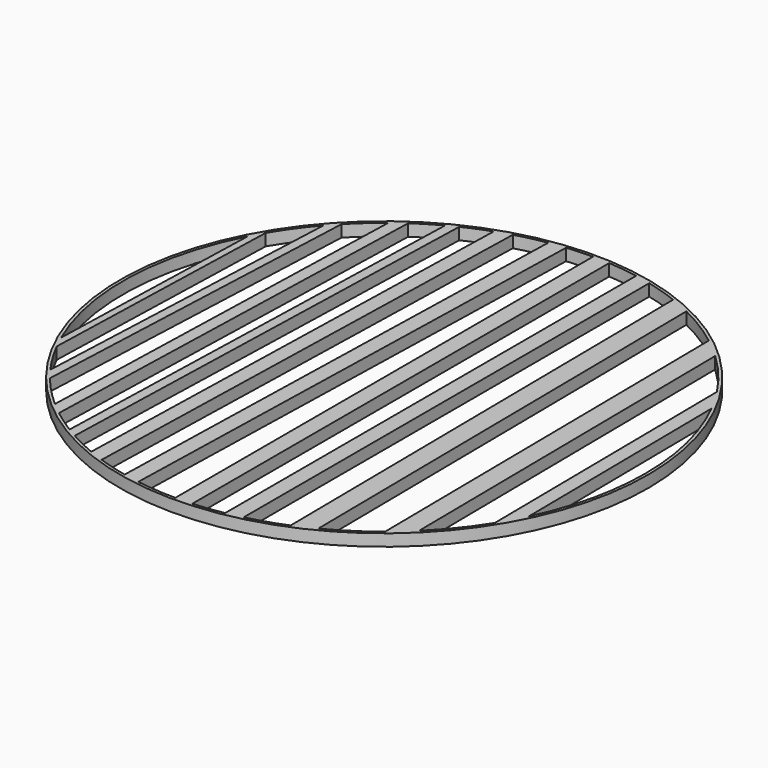
from build123d import *

# Parameters (mm, degrees)
F1_DEPTH = 20


with BuildPart() as f1:
    # F0 (on Top) → F1 (new body)
    with BuildSketch(Plane.XY):
        with BuildLine():
            Line((-270.5386970375, -346.9997311313), (-270.7217620056, -353.178039488))
            ThreePointArc((-270.7217620056, -353.178039488), (-250.9562000988, -367.4860346081), (-230.4360952891, -380.6891198707))
            Line((-230.4360952891, -380.6891198707), (-230.265657339, -374.9369641023))
            ThreePointArc((-230.2656573389, -374.9369641023), (-250.7914922543, -361.5295664436), (-270.5386970375, -346.9997311313))
        make_face()
        with BuildLine():
            ThreePointArc((-402.562994487, -177.6035908131), (-397.2206510106, -189.250507029), (-391.5414264828, -200.7369207392))
            Line((-391.5414264828, -200.7369207392), (-378.8101580312, 223.8366908537))
            ThreePointArc((-378.8101580312, 223.8366908537), (-385.1674232463, 212.7112034422), (-391.1980296982, 201.4053166136))
            Line((-391.1980296982, 201.4053166136), (-402.562994487, -177.6035908131))
        make_face()
        with BuildLine():
            ThreePointArc((-356.5130720875, -257.8728939433), (-349.3185745571, -267.5379103406), (-341.8621362052, -277.0023101514))
            Line((-341.8621362052, -277.0023101514), (-316.4372711676, 305.7244730407))
            ThreePointArc((-316.4372711676, 305.7244730407), (-324.6896849683, 296.9454638064), (-332.6986262228, 287.9437863707))
            Line((-332.6986262228, 287.9437863707), (-356.5130720875, -257.8728939433))
        make_face()
        with BuildLine():
            ThreePointArc((-290.771309932, -330.2302913429), (-280.7802245685, -338.7660925938), (-270.5386970375, -346.9997311313))
            Line((-270.5386970375, -346.9997311313), (-249.5187169425, 362.4091746843))
            ThreePointArc((-249.5187169425, 362.4091746843), (-260.22977901, 354.7963671127), (-270.708728898, 346.8670986105))
            Line((-270.708728898, 346.8670986105), (-290.771309932, -330.2302913429))
        make_face()
        with BuildLine():
            Line((-207.6622074156, 387.912886627), (-230.265657339, -374.9369641023))
            ThreePointArc((-230.2656573389, -374.9369641023), (-222.1173118779, -379.8208785258), (-213.8654246951, -384.5277364768))
            Line((-213.8654246951, -384.5277364768), (-190.7228909108, 396.5157990328))
            ThreePointArc((-190.7228909108, 396.5157990328), (-199.2389875692, 392.3057810336), (-207.6622074156, 387.912886627))
        make_face()
        with BuildLine():
            Line((-70.8738586956, 434.2544140865), (-70.7405367429, 439.341298379))
            ThreePointArc((-70.7405367429, 439.341298379), (-431.4752027521, 108.8767624889), (-270.7217620056, -353.178039488))
            Line((-270.7217620056, -353.178039488), (-270.5386970375, -346.9997311313))
            ThreePointArc((-270.5386970375, -346.9997311313), (-280.7802245685, -338.7660925938), (-290.771309932, -330.2302913429))
            ThreePointArc((-290.771309932, -330.2302913429), (-317.4343613856, -304.6890648049), (-341.8621362052, -277.0023101514))
            ThreePointArc((-341.8621362052, -277.0023101514), (-349.3185745571, -267.5379103406), (-356.5130720875, -257.8728939433))
            ThreePointArc((-356.5130720875, -257.8728939433), (-375.1166659405, -229.9727960731), (-391.5414264828, -200.7369207392))
            ThreePointArc((-391.5414264828, -200.7369207392), (-397.2206510106, -189.250507029), (-402.562994487, -177.6035908131))
            ThreePointArc((-402.562994487, -177.6035908131), (-439.8023179294, 13.187916588), (-391.1980296982, 201.4053166136))
            ThreePointArc((-391.1980296982, 201.4053166136), (-385.1674232463, 212.7112034422), (-378.8101580312, 223.8366908537))
            ThreePointArc((-378.8101580312, 223.8366908537), (-357.1954891114, 256.9268038926), (-332.6986262228, 287.9437863707))
            ThreePointArc((-332.6986262228, 287.9437863707), (-324.6896849683, 296.9454638064), (-316.4372711676, 305.7244730407))
            ThreePointArc((-316.4372711676, 305.7244730407), (-294.2928562808, 327.0958800445), (-270.708728898, 346.8670986105))
            ThreePointArc((-270.708728898, 346.8670986105), (-260.22977901, 354.7963671127), (-249.5187169425, 362.4091746843))
            ThreePointArc((-249.5187169425, 362.4091746843), (-228.9458652825, 375.7443156856), (-207.6622074156, 387.912886627))
            ThreePointArc((-207.6622074156, 387.912886627), (-199.2389875692, 392.3057810336), (-190.7228909108, 396.5157990328))
            ThreePointArc((-190.7228909108, 396.5157990328), (-169.0852127848, 406.2144640673), (-146.9564772982, 414.7334008494))
            ThreePointArc((-146.9564772982, 414.7334008494), (-134.2564645291, 419.0169468317), (-121.4318768159, 422.9116920741))
            ThreePointArc((-121.4318768159, 422.9116920741), (-96.3199787859, 429.3279185968), (-70.8738586956, 434.2544140865))
        make_face()
        with BuildLine():
            Line((-143.4181009985, -415.9702493039), (-121.4318768159, 422.9116920741))
            ThreePointArc((-121.4318768159, 422.9116920741), (-134.2564645291, 419.0169468317), (-146.9564772982, 414.7334008494))
            Line((-146.9564772982, 414.7334008494), (-168.4792645982, -406.4661577554))
            ThreePointArc((-168.4792645982, -406.4661577554), (-156.0210678261, -411.4090742733), (-143.4181009985, -415.9702493039))
        make_face()
        with BuildLine():
            ThreePointArc((-43.616286433, 437.8328671511), (-57.2730273731, 436.2565762662), (-70.8738586956, 434.2544140865))
            Line((-70.8738586956, 434.2544140865), (-93.5236465706, -429.9457262634))
            ThreePointArc((-93.5236465706, -429.9457262634), (-80.0463646466, -432.6575776603), (-66.4909418972, -434.9470710852))
            Line((-66.4909418972, -434.9470710852), (-43.616286433, 437.8328671511))
        make_face()
        with BuildLine():
            Line((0, 440), (0, -440))
            ThreePointArc((0, -440), (14.0186355194, -439.7766226827), (28.0230371971, -439.1067175372))
            Line((28.0230371971, -439.1067175372), (28.0230371971, 439.1067175372))
            ThreePointArc((28.0230371971, 439.1067175372), (14.0186355194, 439.7766226827), (0, 440))
        make_face()
        with BuildLine():
            Line((78.35839003, 432.9664683459), (78.35839003, -432.9664683459))
            ThreePointArc((78.35839003, -432.9664683459), (91.7286409393, -430.3322628289), (105.0109050122, -427.2852792088))
            Line((105.0109050122, -427.2852792088), (105.0109050122, 427.2852792088))
            ThreePointArc((105.0109050122, 427.2852792088), (91.7286409393, 430.3322628289), (78.35839003, 432.9664683459))
        make_face()
        with BuildLine():
            Line((158.8886932936, 410.3101060704), (167.7992454591, -406.7473579796))
            ThreePointArc((167.7992454591, -406.7473579796), (184.9665523772, -399.233483693), (201.798344937, -390.9954321737))
            Line((201.798344937, -390.9954321737), (193.2232359584, 395.3034038378))
            ThreePointArc((193.2232359584, 395.3034038378), (176.2157852134, 403.1724160228), (158.8886932936, 410.3101060704))
        make_face()
        with BuildLine():
            Line((268.376457209, 348.6747441613), (275.9167800325, -342.7388663348))
            ThreePointArc((275.9167800325, -342.7388663348), (292.9545944223, -328.2949978402), (309.2374568684, -313.0051042228))
            Line((309.2374568684, -313.0051042228), (302.3376646701, 319.6747355075))
            ThreePointArc((302.3376646701, 319.6747355075), (285.7252217666, 334.6058840583), (268.376457209, 348.6747441613))
        make_face()
        with BuildLine():
            Line((367.9772639554, 241.2317002633), (373.1507016006, -233.1492095096))
            ThreePointArc((373.1507016006, -233.1492095096), (385.3711791661, -212.3418335329), (396.4325833067, -190.8958011398))
            Line((396.4325833067, -190.8958011398), (392.175101476, 199.4960896417))
            ThreePointArc((392.175101476, 199.4960896417), (380.6486174495, 220.6957861714), (367.9772639554, 241.2317002633))
        make_face()
        with BuildLine():
            ThreePointArc((0, -445), (314.662517628, -314.662517628), (445, 0))
            ThreePointArc((445, 0), (288.570148447, 338.7510434306), (-70.7405367429, 439.341298379))
            Line((-70.7405367429, 439.341298379), (-70.8738586956, 434.2544140865))
            ThreePointArc((-70.8738586956, 434.2544140865), (-57.2730273731, 436.2565762662), (-43.616286433, 437.8328671511))
            ThreePointArc((-43.616286433, 437.8328671511), (-21.835045838, 439.4578828207), (0, 440))
            ThreePointArc((0, 440), (14.0186355194, 439.7766226827), (28.0230371971, 439.1067175372))
            ThreePointArc((28.0230371971, 439.1067175372), (53.2792424848, 436.7623178804), (78.35839003, 432.9664683459))
            ThreePointArc((78.35839003, 432.9664683459), (91.7286409393, 430.3322628289), (105.0109050122, 427.2852792088))
            ThreePointArc((105.0109050122, 427.2852792088), (132.2224966571, 419.663211847), (158.8886932936, 410.3101060704))
            ThreePointArc((158.8886932936, 410.3101060704), (176.2157852134, 403.1724160228), (193.2232359584, 395.3034038378))
            ThreePointArc((193.2232359584, 395.3034038378), (231.9744105691, 373.8821643795), (268.376457209, 348.6747441613))
            ThreePointArc((268.376457209, 348.6747441613), (285.7252217666, 334.6058840583), (302.3376646701, 319.6747355075))
            ThreePointArc((302.3376646701, 319.6747355075), (337.4445929766, 282.3670424658), (367.9772639554, 241.2317002633))
            ThreePointArc((367.9772639554, 241.2317002633), (380.6486174495, 220.6957861714), (392.175101476, 199.4960896417))
            ThreePointArc((392.175101476, 199.4960896417), (427.8767606738, 102.5742544467), (440, 0))
            ThreePointArc((440, 0), (428.969892099, -97.9021535643), (396.4325833067, -190.8958011398))
            ThreePointArc((396.4325833067, -190.8958011398), (385.3711791661, -212.3418335329), (373.1507016006, -233.1492095096))
            ThreePointArc((373.1507016006, -233.1492095096), (343.5224020131, -274.9406468952), (309.2374568684, -313.0051042228))
            ThreePointArc((309.2374568684, -313.0051042228), (292.9545944223, -328.2949978402), (275.9167800325, -342.7388663348))
            ThreePointArc((275.9167800325, -342.7388663348), (240.0731330091, -368.7341736362), (201.798344937, -390.9954321737))
            ThreePointArc((201.798344937, -390.9954321737), (184.9665523772, -399.233483693), (167.7992454591, -406.7473579796))
            ThreePointArc((167.7992454591, -406.7473579796), (136.7910673332, -418.1963700199), (105.0109050122, -427.2852792088))
            ThreePointArc((105.0109050122, -427.2852792088), (91.7286409393, -430.3322628289), (78.35839003, -432.9664683459))
            ThreePointArc((78.35839003, -432.9664683459), (53.2792424848, -436.7623178804), (28.0230371971, -439.1067175372))
            ThreePointArc((28.0230371971, -439.1067175372), (14.0186355194, -439.7766226827), (0, -440))
            Line((0, -440), (0, -445))
        make_face()
        with BuildLine():
            ThreePointArc((-230.4360952891, -380.6891198707), (-119.6209464466, -428.6208454698), (0, -445))
            Line((0, -445), (0, -440))
            ThreePointArc((0, -440), (-33.3413311259, -438.7349491877), (-66.4909418972, -434.9470710852))
            ThreePointArc((-66.4909418972, -434.9470710852), (-80.0463646466, -432.6575776603), (-93.5236465706, -429.9457262634))
            ThreePointArc((-93.5236465706, -429.9457262634), (-118.6767728932, -423.693077092), (-143.4181009985, -415.9702493039))
            ThreePointArc((-143.4181009985, -415.9702493039), (-156.0210678261, -411.4090742733), (-168.4792645982, -406.4661577554))
            ThreePointArc((-168.4792645982, -406.4661577554), (-191.4867852876, -396.1474612568), (-213.8654246951, -384.5277364768))
            ThreePointArc((-213.8654246951, -384.5277364768), (-222.1173118779, -379.8208785258), (-230.2656573389, -374.9369641023))
            Line((-230.265657339, -374.9369641023), (-230.4360952891, -380.6891198707))
        make_face()
    extrude(amount=-F1_DEPTH)


solid = f1.part
